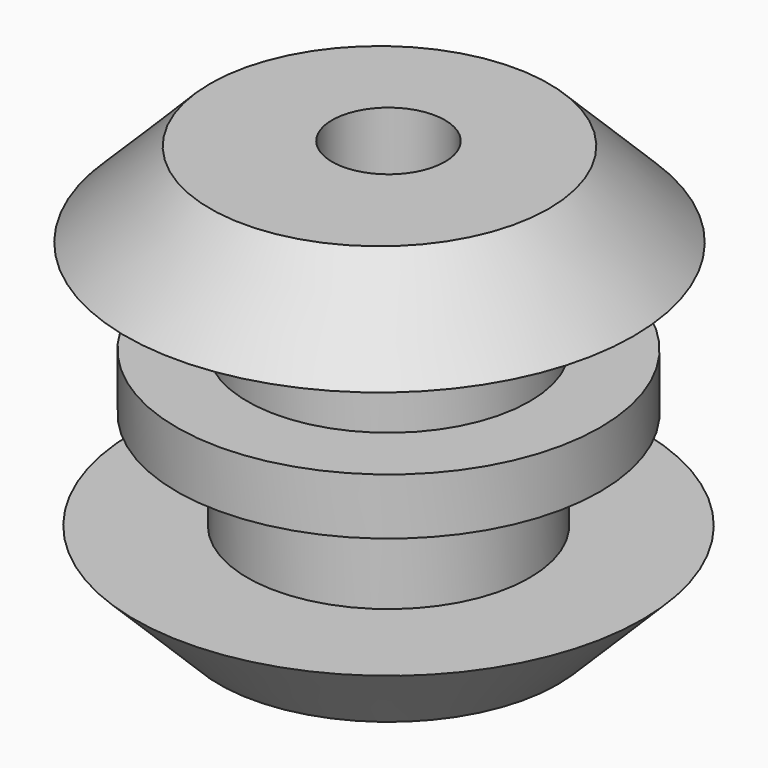
from build123d import *

# Parameters (mm, degrees)
F0_R      = 12.7
F1_DEPTH  = 3.81
F2_R      = 6.35
F3_DEPTH  = 4.445
F4_R      = 9.525
F5_DEPTH  = 2.54
F6_R      = 6.35
F7_DEPTH  = 4.445
F8_R      = 12.7
F9_DEPTH  = 3.81
F10_R     = 2.54
F11_DEPTH = 19.05


# Not quite as in the source:
# - a fillet or chamfer that OpenCascade refuses, or shapes differently, is made with other operations: its cross-section is extruded or revolved along the edge and cut away or added


with BuildPart() as f1:
    # F0 (on Top) → F1 (new body)
    with BuildSketch(Plane.XY):
        Circle(F0_R)
    extrude(amount=F1_DEPTH)

    # F2 (on face) → F3 (join)
    with BuildSketch(Plane.XY.offset(3.81)):
        Circle(F2_R)
    extrude(amount=F3_DEPTH)

    # F4 (on face) → F5 (join)
    with BuildSketch(Plane.XY.offset(8.255)):
        Circle(F4_R)
    extrude(amount=F5_DEPTH)

    # F6 (on face) → F7 (join)
    with BuildSketch(Plane.XY.offset(10.795)):
        Circle(F6_R)
    extrude(amount=F7_DEPTH)

    # F8 (on face) → F9 (join)
    with BuildSketch(Plane.XY.offset(15.24)):
        with Locations((0, -0.5063372408)):
            Circle(F8_R)
    extrude(amount=F9_DEPTH)

    # F10 (on face) → F11 (cut)
    with BuildSketch(Plane.XY.offset(19.05)):
        Circle(F10_R)
    extrude(amount=-F11_DEPTH, mode=Mode.SUBTRACT)

    # F12: chamfer of 5.08 on 1 edges, made by hand

    # F12_s1 → F12_t2 (revolve, cut)
    with BuildSketch(Plane.XZ.offset(0.5063372408)):
        Polygon((12.7, 13.97), (7.62, 19.05), (12.7, 19.05), align=None)
    revolve(axis=Axis((0, -0.5063372408, 19.05), (0, 0, 1)), mode=Mode.SUBTRACT)

    # F13: chamfer of 5.08 on 1 edges, made by hand

    # F13_s1 → F13_t2 (revolve, cut)
    with BuildSketch(Plane.XZ):
        Polygon((7.62, 0), (12.7, 5.08), (12.7, 0), align=None)
    revolve(axis=Axis((0, 0, 0), (0, 0, 1)), mode=Mode.SUBTRACT)


solid = f1.part
